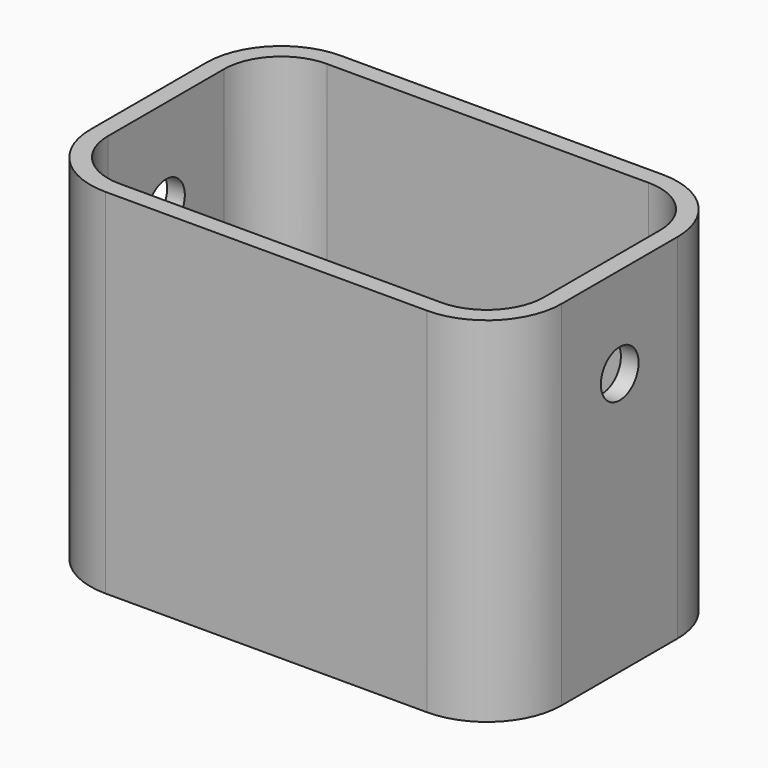
from build123d import *

# Parameters (mm, degrees)
F0_W     = 80
F0_H     = 50
F1_DEPTH = 60
F2_R     = 12.7
F3_T     = -3
F5_D     = 8


# Not quite as in the source:
# - a feature names something its author has since deleted; it is built from what else it names


with BuildPart() as f1:
    # F0 (on Top) → F1 (new body)
    with BuildSketch(Plane.XY):
        with Locations((-2.1280694621, 0)):
            Rectangle(F0_W, F0_H)
    extrude(amount=F1_DEPTH)

    # F2
    f2_edges = [f1.edges().sort_by_distance(p)[0] for p in [
        (-42.128069, -25, 30),
        (37.871931, 25, 30),
        (37.871931, -25, 30),
        (-42.128069, 25, 30),
    ]]
    fillet(f2_edges, radius=F2_R)

    # F3
    f3_openings = [f1.faces().sort_by_distance(p)[0] for p in [
        (-2.128069, 0, 60),
    ]]
    offset(amount=F3_T, openings=f3_openings)

    # F5 (through all)
    with Locations(Plane.YZ.offset(37.8719305379)):
        with Locations((0, 44.5649288595)):
            Hole(F5_D / 2)


solid = f1.part
